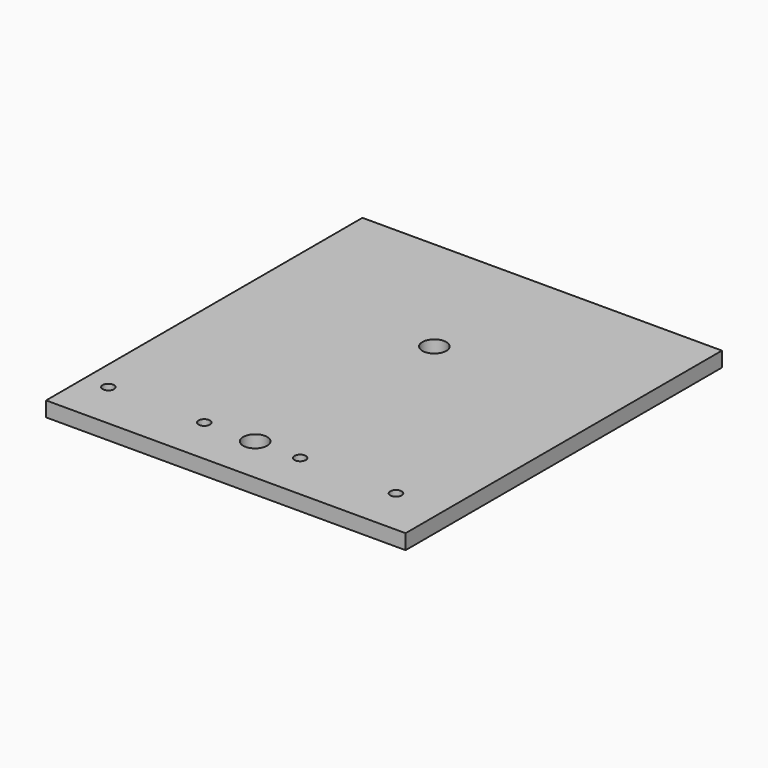
from build123d import *

# Parameters (mm, degrees)
F0_W     = 120
F0_H     = 132
F0_R     = 1.9
F0_R_2   = 4
F1_DEPTH = 5
F2_R     = 4
F3_DEPTH = 25


# Not quite as in the source:
# - a feature names something its author has since deleted; it is built from what else it names


with BuildPart() as f1:
    # F0 (on Top) → F1 (new body)
    with BuildSketch(Plane.XY):
        Rectangle(F0_W, F0_H)
        with Locations((-52, -50)):
            Circle(F0_R, mode=Mode.SUBTRACT)
        with Locations((-20, -50)):
            Circle(F0_R, mode=Mode.SUBTRACT)
        with Locations((-3, -50)):
            Circle(F0_R_2, mode=Mode.SUBTRACT)
        with Locations((12, -50)):
            Circle(F0_R, mode=Mode.SUBTRACT)
        with Locations((44, -50)):
            Circle(F0_R, mode=Mode.SUBTRACT)
    extrude(amount=F1_DEPTH)

    # F2 (on face) → F3 (cut)
    with BuildSketch(Plane.XY.offset(5)):
        with Locations((0, 21)):
            Circle(F2_R)
    extrude(amount=-F3_DEPTH, mode=Mode.SUBTRACT)


solid = f1.part
